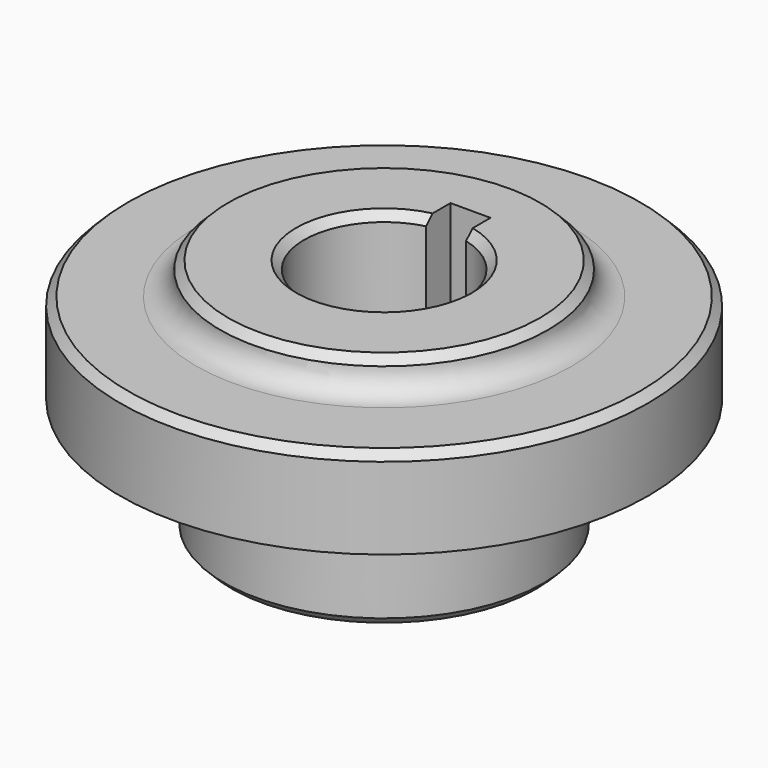
from build123d import *

# Parameters (mm, degrees)
F2_SIZE  = 1
F3_R     = 2.99999
F5_DEPTH = 30


# Not quite as in the source:
# - a fillet or chamfer is up to 0.001 mm smaller than in the source, because OpenCascade refuses the exact size


with BuildPart() as f1:
    # F0 (on Front) → F1 (revolve)
    with BuildSketch(Plane.XZ):
        Polygon((10, 30), (10, 0), (20, 0), (20, 14), (28.5, 14), (33, 14.7934714132), (33, 26), (20.5, 26), (20.5, 30), align=None)
    revolve(axis=Axis((0, 0, 2.9418331105), (0, 0, 1)))

    # F2
    f2_edges = [f1.edges().sort_by_distance(p)[0] for p in [
        (-20.5, 0, 30),
        (-33, 0, 26),
        (-20, 0, 0),
        (-10, 0, 30),
        (-10, 0, 0),
    ]]
    chamfer(f2_edges, length=F2_SIZE)

    # F3 (radius 3 in the source; OpenCascade refuses exactly that, so slightly less here)
    f3_edges = [f1.edges().sort_by_distance(p)[0] for p in [
        (-20, 0, 14),
        (-20.5, 0, 26),
    ]]
    fillet(f3_edges, radius=F3_R)

    # F4 (on face) → F5 (cut, through all)
    with BuildSketch(Plane.XY.offset(30)):
        with BuildLine():
            Line((2.5, 13.5), (-2.5, 13.5))
            Line((-2.5, 13.5), (-2.5, 10.7121426428))
            ThreePointArc((-2.5, 10.7121426428), (0, 11), (2.5, 10.7121426428))
            Line((2.5, 10.7121426428), (2.5, 13.5))
        make_face()
        with BuildLine():
            ThreePointArc((2.5, 10.7121426428), (0, 11), (-2.5, 10.7121426428))
            Line((-2.5, 10.7121426428), (-2.5, 9.6824583655))
            ThreePointArc((-2.5, 9.6824583655), (0, 10), (2.5, 9.6824583655))
            Line((2.5, 9.6824583655), (2.5, 10.7121426428))
        make_face()
    extrude(amount=-F5_DEPTH, mode=Mode.SUBTRACT)


solid = f1.part
